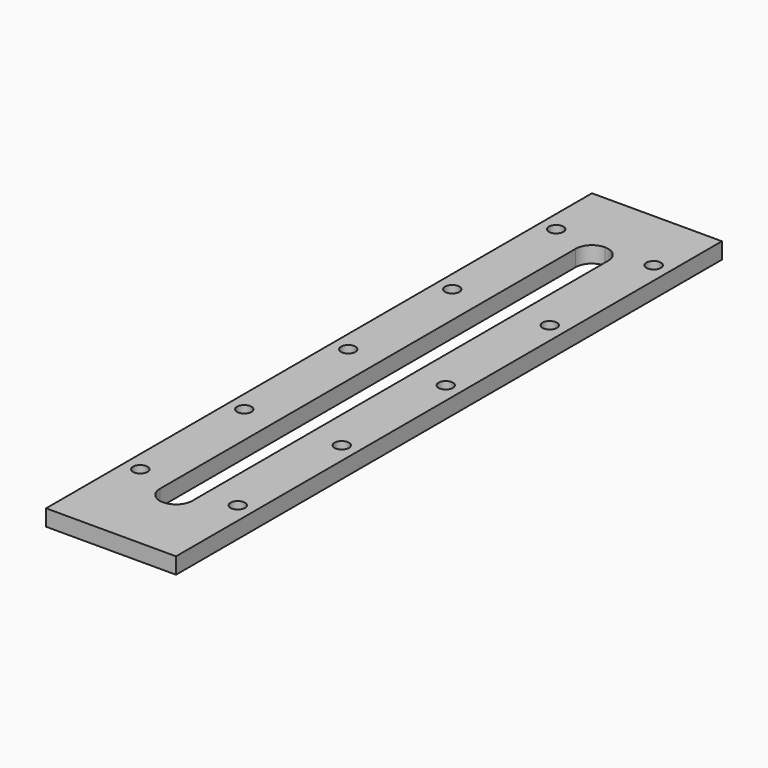
from build123d import *

# Parameters (mm, degrees)
F0_W          = 40
F0_H          = 210
F0_R          = 2.2155
F0_W_2        = 10
F0_H_2        = 170
F1_DEPTH      = 2.5
F1_DEPTH_BACK = 2.5
F2_R          = 4.99999


# Not quite as in the source:
# - a fillet or chamfer is up to 0.001 mm smaller than in the source, because OpenCascade refuses the exact size


with BuildPart() as f1:
    # F0 (on Top) → F1 (new body, two sides)
    with BuildSketch(Plane.XY) as f1_sk:
        Rectangle(F0_W, F0_H)
        with Locations((-15, -75)):
            Circle(F0_R, mode=Mode.SUBTRACT)
        with Locations((-15, -35)):
            Circle(F0_R, mode=Mode.SUBTRACT)
        with Locations((15, -75)):
            Circle(F0_R, mode=Mode.SUBTRACT)
        with Locations((15, -35)):
            Circle(F0_R, mode=Mode.SUBTRACT)
        with Locations((-15, 5)):
            Circle(F0_R, mode=Mode.SUBTRACT)
        with Locations((-15, 45)):
            Circle(F0_R, mode=Mode.SUBTRACT)
        with Locations((-15, 85)):
            Circle(F0_R, mode=Mode.SUBTRACT)
        Rectangle(F0_W_2, F0_H_2, mode=Mode.SUBTRACT)
        with Locations((15, 5)):
            Circle(F0_R, mode=Mode.SUBTRACT)
        with Locations((15, 45)):
            Circle(F0_R, mode=Mode.SUBTRACT)
        with Locations((15, 85)):
            Circle(F0_R, mode=Mode.SUBTRACT)
    extrude(amount=F1_DEPTH)
    extrude(f1_sk.sketch, amount=-F1_DEPTH_BACK)

    # F2 (radius 5 in the source; OpenCascade refuses exactly that, so slightly less here)
    f2_edges = [f1.edges().sort_by_distance(p)[0] for p in [
        (-5, 85, 0),
        (5, 85, 0),
        (-5, -85, 0),
        (5, -85, 0),
    ]]
    fillet(f2_edges, radius=F2_R)


solid = f1.part
